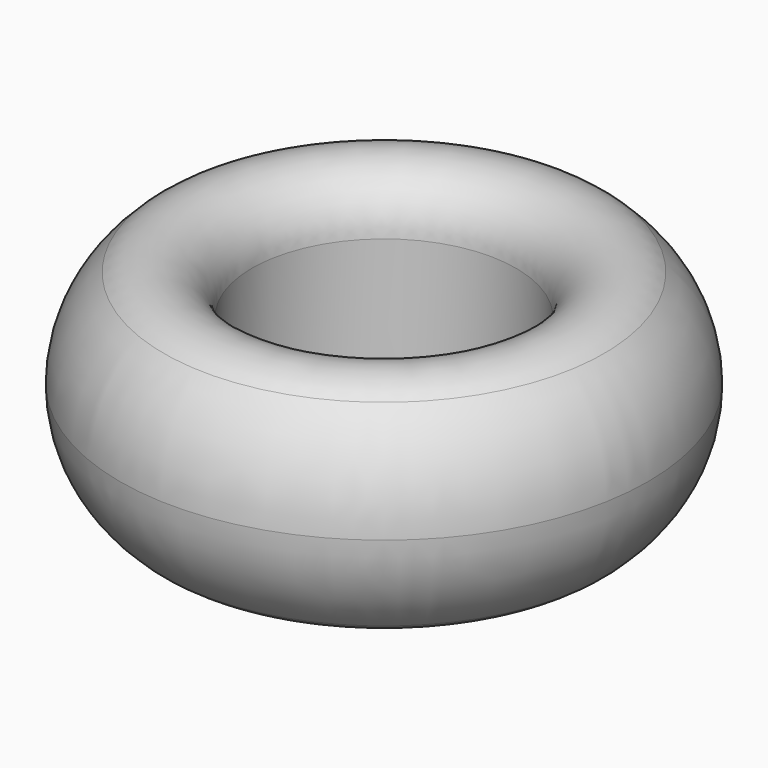
from build123d import *

# Parameters (mm, degrees)
F0_W     = 1270
F0_H     = 1270
F2_R     = 634.99999
F3_DEPTH = 1270.001
F4_R     = 254


# Not quite as in the source:
# - a fillet or chamfer is up to 0.001 mm smaller than in the source, because OpenCascade refuses the exact size


with BuildPart() as f1:
    # F0 (on Front) → F1 (revolve)
    with BuildSketch(Plane.XZ):
        with Locations((-635, 635)):
            Rectangle(F0_W, F0_H)
    revolve(axis=Axis((0, 0, 635), (0, 0, 1)))

    # F2 (radius 635 in the source; OpenCascade refuses exactly that, so slightly less here)
    f2_edges = [f1.edges().sort_by_distance(p)[0] for p in [
        (1270, 0, 1270),
        (1270, 0, 0),
        (-1270, 0, 635),
    ]]
    fillet(f2_edges, radius=F2_R)

    # F3 (cut, through all): a face of the model
    f3_faces = [f1.faces().sort_by_distance(p)[0] for p in [
        (0, 0, 1270),
    ]]
    extrude(f3_faces, amount=-F3_DEPTH, mode=Mode.SUBTRACT)

    # F4
    f4_edges = [f1.edges().sort_by_distance(p)[0] for p in [
        (635.00001, 0, 1270),
        (635.00001, 0, 0),
    ]]
    fillet(f4_edges, radius=F4_R)


solid = f1.part
